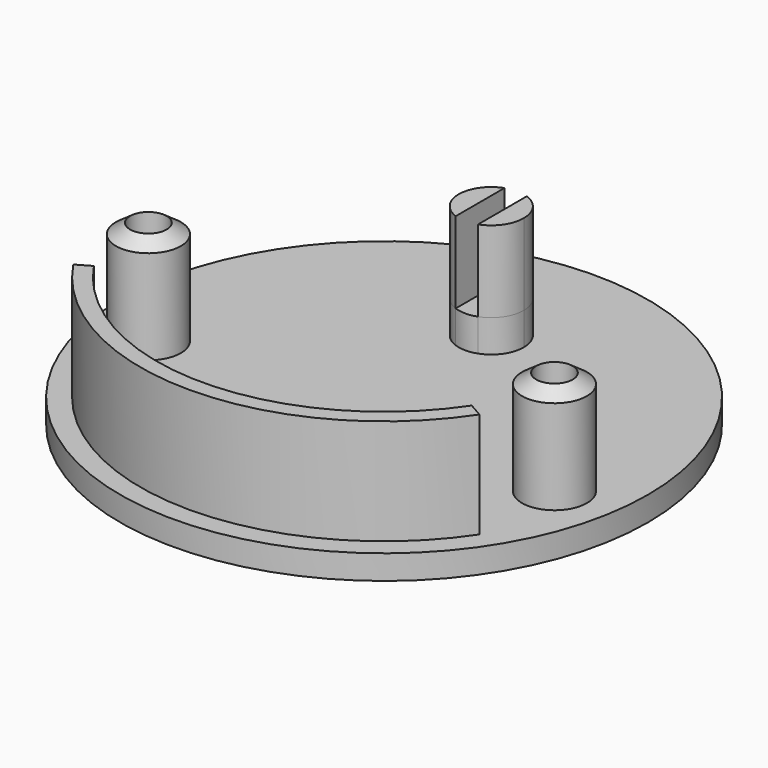
from build123d import *
from build123d import SkipClean  # not in build123d's __all__

# Parameters (mm, degrees)
F0_R     = 32.5
F0_R_2   = 4
F0_R_3   = 2.25
F1_DEPTH = 3
F2_START = 3
F2_DEPTH = 13
F3_START = 3
F3_DEPTH = 13
F5_START = 3
F5_DEPTH = 4
F6_START = 7
F6_DEPTH = 10


# Not quite as in the source:
# - a fillet or chamfer that OpenCascade refuses, or shapes differently, is made with other operations: its cross-section is extruded or revolved along the edge and cut away or added


with BuildPart() as f1:
    # F0 (on Top) → F1 (new body)
    with BuildSketch(Plane.XY):
        Circle(F0_R)
        with Locations((-25, -5.0249378106)):
            Circle(F0_R_2, mode=Mode.SUBTRACT)
        with BuildLine():
            ThreePointArc((25, -16.5831239518), (0, -30), (-25, -16.5831239518))
            Line((-25, -16.5831239518), (-23.2643659014, -15.5810551377))
            Line((-23.2643659014, -15.5810551377), (23.2643659014, -15.5810551377))
            Line((23.2643659014, -15.5810551377), (25, -16.5831239518))
        make_face(mode=Mode.SUBTRACT)
        with Locations((25, -5.0249378106)):
            Circle(F0_R_2, mode=Mode.SUBTRACT)
        with BuildLine():
            ThreePointArc((1.375, 20.2562448003), (3.2787192622, 18.7912878475), (4, 16.5))
            ThreePointArc((4, 16.5), (3.2787192622, 14.2087121525), (1.375, 12.7437551997))
            ThreePointArc((1.375, 12.7437551997), (0, 12.5), (-1.375, 12.7437551997))
            ThreePointArc((-1.375, 12.7437551997), (-4, 16.5), (-1.375, 20.2562448003))
            ThreePointArc((-1.375, 20.2562448003), (0, 20.5), (1.375, 20.2562448003))
        make_face(mode=Mode.SUBTRACT)
        with BuildLine():
            Line((23.2643659014, -15.5810551377), (-23.2643659014, -15.5810551377))
            ThreePointArc((-23.2643659014, -15.5810551377), (0, -28), (23.2643659014, -15.5810551377))
        make_face()
        with BuildLine():
            Line((-23.2643659014, -15.5810551377), (-25, -16.5831239518))
            ThreePointArc((-25, -16.5831239518), (0, -30), (25, -16.5831239518))
            Line((25, -16.5831239518), (23.2643659014, -15.5810551377))
            ThreePointArc((23.2643659014, -15.5810551377), (0, -28), (-23.2643659014, -15.5810551377))
        make_face()
        with Locations((25, -5.0249378106)):
            Circle(F0_R_2)
        with Locations((25, -5.0249378106)):
            Circle(F0_R_3, mode=Mode.SUBTRACT)
        with Locations((-25, -5.0249378106)):
            Circle(F0_R_2)
        with Locations((-25, -5.0249378106)):
            Circle(F0_R_3, mode=Mode.SUBTRACT)
        with BuildLine():
            Line((1.375, 12.7437551997), (1.375, 20.2562448003))
            ThreePointArc((1.375, 20.2562448003), (0, 20.5), (-1.375, 20.2562448003))
            Line((-1.375, 20.2562448003), (-1.375, 12.7437551997))
            ThreePointArc((-1.375, 12.7437551997), (0, 12.5), (1.375, 12.7437551997))
        make_face()
        with Locations((25, -5.0249378106)):
            Circle(F0_R_3)
        with Locations((-25, -5.0249378106)):
            Circle(F0_R_3)
        with BuildLine():
            ThreePointArc((1.375, 12.7437551997), (3.2787192622, 14.2087121525), (4, 16.5))
            ThreePointArc((4, 16.5), (3.2787192622, 18.7912878475), (1.375, 20.2562448003))
            Line((1.375, 20.2562448003), (1.375, 12.7437551997))
        make_face()
        with BuildLine():
            Line((-1.375, 12.7437551997), (-1.375, 20.2562448003))
            ThreePointArc((-1.375, 20.2562448003), (-4, 16.5), (-1.375, 12.7437551997))
        make_face()
    extrude(amount=F1_DEPTH)

    # F0 (on Top) → F2 (join)
    with BuildSketch(Plane.XY.offset(F2_START)):
        with BuildLine():
            Line((-23.2643659014, -15.5810551377), (-25, -16.5831239518))
            ThreePointArc((-25, -16.5831239518), (0, -30), (25, -16.5831239518))
            Line((25, -16.5831239518), (23.2643659014, -15.5810551377))
            ThreePointArc((23.2643659014, -15.5810551377), (0, -28), (-23.2643659014, -15.5810551377))
        make_face()
    extrude(amount=F2_DEPTH)

    # F0 (on Top) → F3 (join)
    with BuildSketch(Plane.XY.offset(F3_START)):
        with Locations((-25, -5.0249378106)):
            Circle(F0_R_2)
        with Locations((-25, -5.0249378106)):
            Circle(F0_R_3, mode=Mode.SUBTRACT)
        with Locations((25, -5.0249378106)):
            Circle(F0_R_2)
        with Locations((25, -5.0249378106)):
            Circle(F0_R_3, mode=Mode.SUBTRACT)
    extrude(amount=F3_DEPTH)

    # F4: chamfer of 2 x 1.4004150764 on 2 edges, made by hand

    # F4_s1 → F4_t2 (revolve, cut)
    with BuildSketch(Plane.XZ.offset(5.0249378106)):
        Polygon((-21, 14.5995849236), (-23, 16), (-21, 16), align=None)
    revolve(axis=Axis((-25, -5.0249378106, 16), (0, 0, 1)), mode=Mode.SUBTRACT)

    # F4_s3 → F4_t4 (revolve, cut)
    with BuildSketch(Plane.XZ.offset(5.0249378106)):
        Polygon((29, 14.5995849236), (27, 16), (29, 16), align=None)
    revolve(axis=Axis((25, -5.0249378106, 16), (0, 0, 1)), mode=Mode.SUBTRACT)

    # F0 (on Top) → F5 (join)
    with BuildSketch(Plane.XY.offset(F5_START)):
        with BuildLine():
            ThreePointArc((1.375, 12.7437551997), (3.2787192622, 14.2087121525), (4, 16.5))
            ThreePointArc((4, 16.5), (3.2787192622, 18.7912878475), (1.375, 20.2562448003))
            Line((1.375, 20.2562448003), (1.375, 12.7437551997))
        make_face()
        with BuildLine():
            Line((-1.375, 12.7437551997), (-1.375, 20.2562448003))
            ThreePointArc((-1.375, 20.2562448003), (-4, 16.5), (-1.375, 12.7437551997))
        make_face()
        with BuildLine():
            Line((1.375, 12.7437551997), (1.375, 20.2562448003))
            ThreePointArc((1.375, 20.2562448003), (0, 20.5), (-1.375, 20.2562448003))
            Line((-1.375, 20.2562448003), (-1.375, 12.7437551997))
            ThreePointArc((-1.375, 12.7437551997), (0, 12.5), (1.375, 12.7437551997))
        make_face()
    extrude(amount=F5_DEPTH)

    # F0 (on Top) → F6 (join)
    with BuildSketch(Plane.XY.offset(F6_START)):
        with BuildLine():
            Line((-1.375, 12.7437551997), (-1.375, 20.2562448003))
            ThreePointArc((-1.375, 20.2562448003), (-4, 16.5), (-1.375, 12.7437551997))
        make_face()
        with BuildLine():
            ThreePointArc((1.375, 12.7437551997), (3.2787192622, 14.2087121525), (4, 16.5))
            ThreePointArc((4, 16.5), (3.2787192622, 18.7912878475), (1.375, 20.2562448003))
            Line((1.375, 20.2562448003), (1.375, 12.7437551997))
        make_face()
    with SkipClean():  # cleaning this boolean's faces spoils the solid; the shape is the same uncleaned
        extrude(amount=F6_DEPTH)


solid = f1.part
